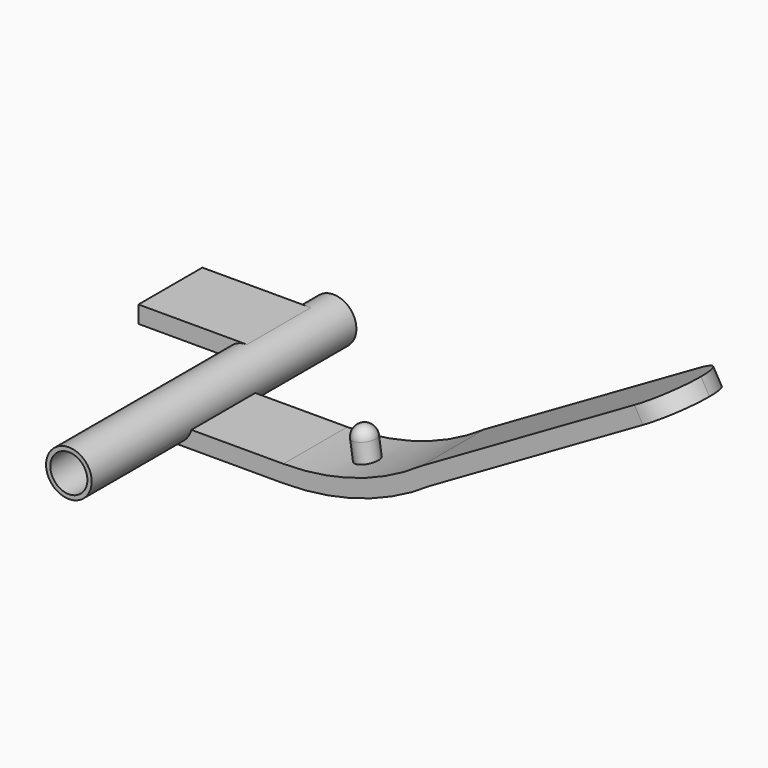
from build123d import *

# Parameters (mm, degrees)
F0_R           = 4
F1_DEPTH       = 58
F2_R           = 3.25
F3_DEPTH       = 13.5
F4_R           = 3.25
F5_DEPTH       = 13.5
F8_DEPTH       = 7
F8_DEPTH_BACK  = 7
F9_R           = 6.99999
F11_W          = 19
F11_H          = 3
F12_DEPTH      = 14
F17_R          = 2
F18_DEPTH      = 5
F18_DEPTH_BACK = 0.471687069
F19_R          = 2


# Not quite as in the source:
# - a fillet or chamfer is up to 0.001 mm smaller than in the source, because OpenCascade refuses the exact size


with BuildPart() as f1:
    # F0 (on Front) → F1 (new body)
    with BuildSketch(Plane.XZ):
        Circle(F0_R)
    extrude(amount=F1_DEPTH)

    # F2 (on face) → F3 (cut)
    with BuildSketch(Plane.XZ.offset(58)):
        Circle(F2_R)
    extrude(amount=-F3_DEPTH, mode=Mode.SUBTRACT)

    # F4 (on face) → F5 (cut)
    with BuildSketch(Plane(origin=(0, 0, 0), x_dir=(-1, 0, 0), z_dir=(0, 1, 0))):
        Circle(F4_R)
    extrude(amount=-F5_DEPTH, mode=Mode.SUBTRACT)

    # F7 (on offset) → F8 (join, two sides)
    with BuildSketch(Plane.XZ.offset(29)) as f8_sk:
        with BuildLine():
            Line((0, -1), (0, -4))
            Line((0, -4), (20, -4))
            ThreePointArc((20, -4), (33.4977869164, -1.9540489613), (45.7829596161, 4))
            Line((45.7829596161, 4), (89.0842298053, 29))
            Line((89.0842298053, 29), (87.5842298053, 31.5980762114))
            Line((87.5842298053, 31.5980762114), (44.1796846254, 6.5384503677))
            ThreePointArc((44.1796846254, 6.5384503677), (32.6637808585, 0.9283092986), (20, -1))
            Line((20, -1), (0, -1))
        make_face()
    extrude(amount=F8_DEPTH)
    extrude(f8_sk.sketch, amount=-F8_DEPTH_BACK)

    # F9 (radius 7 in the source; OpenCascade refuses exactly that, so slightly less here)
    f9_edges = [f1.edges().sort_by_distance(p)[0] for p in [
        (88.33423, -36, 30.299038),
        (88.33423, -22, 30.299038),
    ]]
    fillet(f9_edges, radius=F9_R)

    # F11 (on offset) → F12 (join)
    with BuildSketch(Plane(origin=(0, -5, 0), x_dir=(-1, 0, 0), z_dir=(0, 1, 0))):
        with Locations((9.5, 2.5)):
            Rectangle(F11_W, F11_H)
    extrude(amount=-F12_DEPTH)

    # F17 (on 3pt) → F18 (join, two sides)
    with BuildSketch(Plane(origin=(0.602031742, 0, -3.953721561), x_dir=(0.9886047584, 0, 0.1505344865), z_dir=(-0.1505344865, 0, 0.9886047584))) as f18_sk:
        with Locations((29.0842950344, -29.3515790254)):
            Circle(F17_R)
    extrude(amount=F18_DEPTH)
    extrude(f18_sk.sketch, amount=-F18_DEPTH_BACK)

    # F19
    f19_edges = [f1.edges().sort_by_distance(p)[0] for p in [
        (26.625022, -29.351579, 5.066423),
    ]]
    fillet(f19_edges, radius=F19_R)


solid = f1.part
